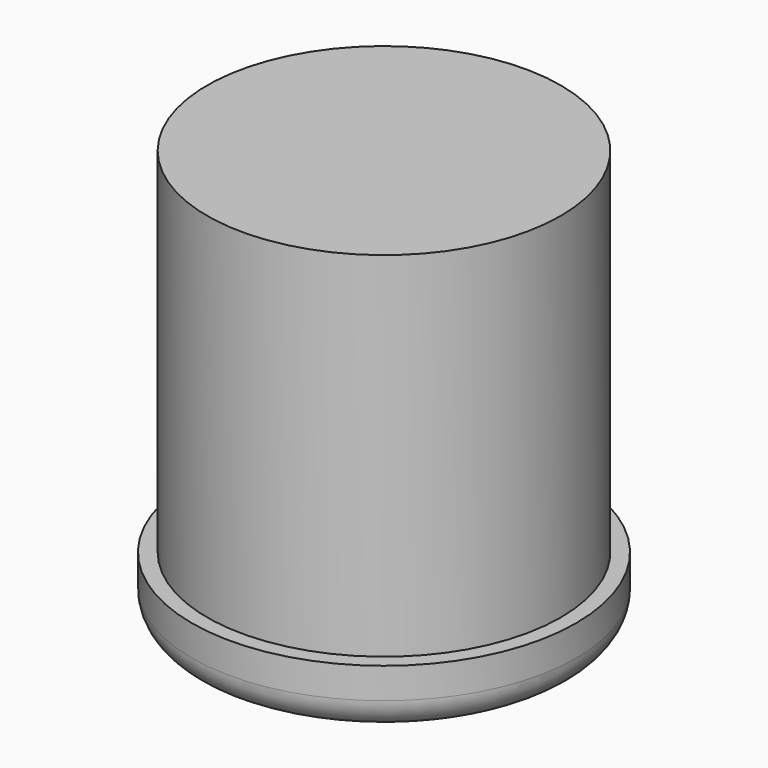
from build123d import *

# Parameters (mm, degrees)
F2_R     = 12.5
F3_DEPTH = 4
F4_R     = 11.5
F5_DEPTH = 23
F6_R     = 2


with BuildPart() as f3:
    # F2 (on Top) → F3 (new body)
    with BuildSketch(Plane.XY):
        Circle(F2_R)
    extrude(amount=F3_DEPTH)

    # F4 (on face) → F5 (join)
    with BuildSketch(Plane.XY.offset(4)):
        Circle(F4_R)
    extrude(amount=F5_DEPTH)

    # F6
    f6_edges = [f3.edges().sort_by_distance(p)[0] for p in [
        (-12.5, 0, 0),
    ]]
    fillet(f6_edges, radius=F6_R)


solid = f3.part
